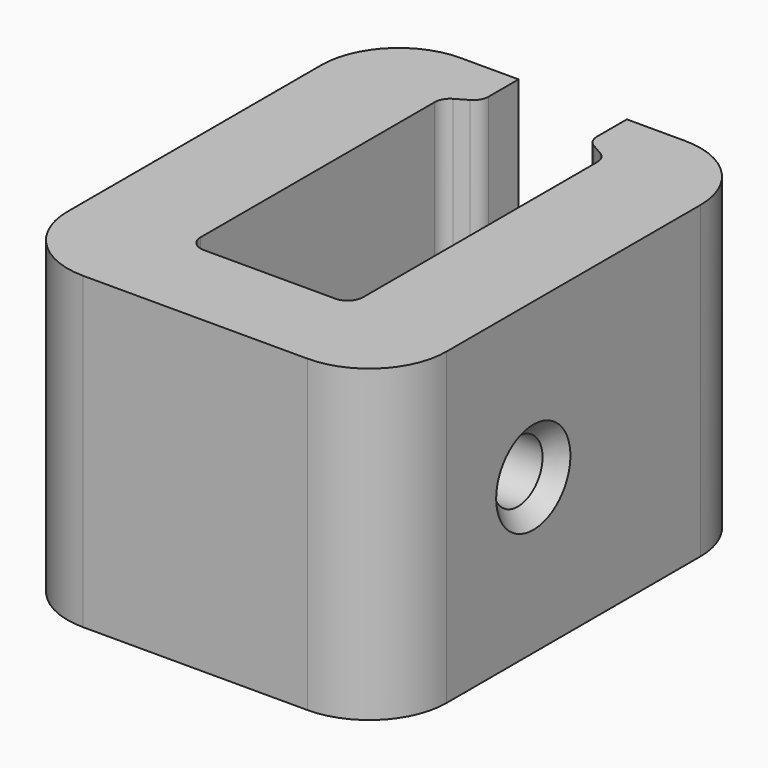
from build123d import *

# Parameters (mm, degrees)
F2_DEPTH = 20
F3_R     = 5
F4_R     = 1
F6_START = -2.5
F6_DEPTH = 7.5
F7_R     = 2
F8_DEPTH = 25
F9_SIZE  = 1
F10_SIZE = 1


# Not quite as in the source:
# - a feature names something its author has since deleted; it is built from what else it names


with BuildPart() as f2:
    # F1 (on Top) → F2 (new body)
    with BuildSketch(Plane.XY):
        Polygon((0.75, 14.5), (-8, 14.5), (-8, -16), (16.5, -16), (16.5, 14.5), (7.75, 14.5), (7.75, 11.5), (9.5, 10.4896370289), (9.5, -10), (-1, -10), (-1, 10.4896370289), (0.75, 11.5), align=None)
    extrude(amount=F2_DEPTH)

    # F3
    f3_edges = [f2.edges().sort_by_distance(p)[0] for p in [
        (-8, 14.5, 10),
        (16.5, 14.5, 10),
        (-8, -16, 10),
        (16.5, -16, 10),
    ]]
    fillet(f3_edges, radius=F3_R)

    # F4
    f4_edges = [f2.edges().sort_by_distance(p)[0] for p in [
        (0.75, 11.5, 10),
        (7.75, 11.5, 10),
        (-1, 10.489637, 10),
        (9.5, 10.489637, 10),
        (9.5, -10, 10),
        (-1, -10, 10),
    ]]
    fillet(f4_edges, radius=F4_R)

    # F5 (on face) → F6 (cut)
    with BuildSketch(Plane.YZ.offset(-1).offset(F6_START)):
        Polygon((-7.897114317, 7.75), (-4, 5.5), (-0.102885683, 7.75), (-0.102885683, 12.25), (-4, 14.5), (-7.897114317, 12.25), align=None)
    extrude(amount=-F6_DEPTH, mode=Mode.SUBTRACT)

    # F7 (on face) → F8 (cut)
    with BuildSketch(Plane(origin=(-3.5, 0, 0), x_dir=(0, -1, 0), z_dir=(-1, 0, 0))):
        with Locations((4, 10)):
            Circle(F7_R)
    extrude(amount=-F8_DEPTH, mode=Mode.SUBTRACT)

    # F9
    f9_edges = [f2.edges().sort_by_distance(p)[0] for p in [
        (-8, -7.897114, 10),
        (-8, -5.948557, 13.375),
        (-8, -2.051443, 13.375),
        (-8, -0.102886, 10),
        (-8, -5.948557, 6.625),
        (-8, -2.051443, 6.625),
    ]]
    chamfer(f9_edges, length=F9_SIZE)

    # F10
    f10_edges = [f2.edges().sort_by_distance(p)[0] for p in [
        (16.5, -2, 10),
        (-1, -2, 10),
        (9.5, -2, 10),
    ]]
    chamfer(f10_edges, length=F10_SIZE)


solid = f2.part
